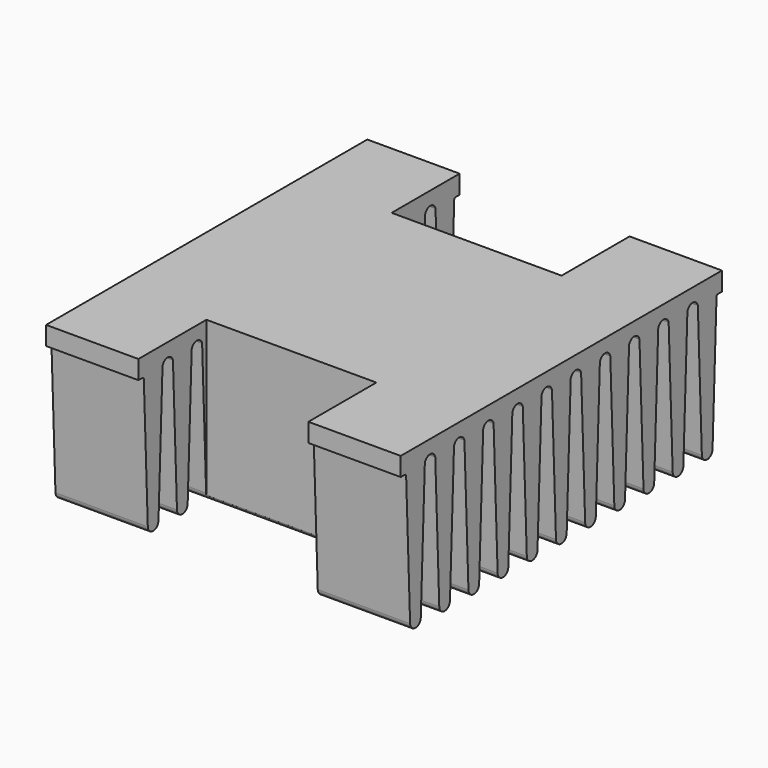
from build123d import *

# Parameters (mm, degrees)
F1_DEPTH = 130
F2_W     = 50.8
F2_H     = 25.4
F3_DEPTH = 79.5
F4_W     = 12
F4_H     = 50.7057624385
F4_H_2   = 69.7820825055
F4_H_3   = 69.8881107867
F4_H_4   = 52.3517530859
F5_DEPTH = 47.4990536315


# Not quite as in the source:
# - ends of sketch curves that miss each other by under 0.0002 mm in the source are joined
# - a feature names something its author has since deleted; it is built from what else it names


with BuildPart() as f1:
    # F0 (on Right) → F1 (new body)
    with BuildSketch(Plane.YZ):
        with BuildLine():
            Line((62.1368927236, 13.271021442), (-57.8631072764, 13.271021442))
            Line((-57.8631072764, 13.271021442), (-57.8631072764, 7.697946392))
            Line((-57.8631072764, 7.697946392), (-56.4219683785, 7.6979366796))
            ThreePointArc((-56.4219683785, 7.6979366796), (-56.0194508606, 7.5356245361), (-55.8421445251, 7.1394791077))
            Line((-55.8421445251, 7.1394791077), (-54.3616227062, -32.302053608))
            ThreePointArc((-54.3616227062, -32.302053608), (-52.3630302548, -34.2270321895), (-50.3644378034, -32.302053608))
            Line((-50.3644378034, -32.302053608), (-48.8631072764, 7.697946392))
            ThreePointArc((-48.8631072764, 7.697946392), (-46.9131019002, 9.2535299318), (-44.9631072764, 7.6979329132))
            Line((-44.9631072764, 7.6979329132), (-43.4616227062, -32.302053608))
            ThreePointArc((-43.4616227062, -32.302053608), (-41.4630302548, -34.2270321895), (-39.4644378034, -32.302053608))
            Line((-39.4644378034, -32.302053608), (-37.9631072764, 7.697946392))
            ThreePointArc((-37.9631072764, 7.697946392), (-36.0131019002, 9.2535299318), (-34.0631072764, 7.6979329132))
            Line((-34.0631072764, 7.6979329132), (-32.5616227062, -32.302053608))
            ThreePointArc((-32.5616227062, -32.302053608), (-30.5630302548, -34.2270321895), (-28.5644378034, -32.302053608))
            Line((-28.5644378034, -32.302053608), (-27.0631072764, 7.697946392))
            ThreePointArc((-27.0631072764, 7.697946392), (-25.1131019002, 9.2535299318), (-23.1631072764, 7.6979329132))
            Line((-23.1631072764, 7.6979329132), (-21.6616227062, -32.302053608))
            ThreePointArc((-21.6616227062, -32.302053608), (-19.6630302548, -34.2270321895), (-17.6644378034, -32.302053608))
            Line((-17.6644378034, -32.302053608), (-16.1631072764, 7.697946392))
            ThreePointArc((-16.1631072764, 7.697946392), (-14.2131019002, 9.2535299318), (-12.2631072764, 7.6979329132))
            Line((-12.2631072764, 7.6979329132), (-10.7616227062, -32.302053608))
            ThreePointArc((-10.7616227062, -32.302053608), (-8.7630302548, -34.2270321895), (-6.7644378034, -32.302053608))
            Line((-6.7644378034, -32.302053608), (-5.2631072764, 7.697946392))
            ThreePointArc((-5.2631072764, 7.697946392), (-3.3131019002, 9.2535299318), (-1.3631072764, 7.6979329132))
            Line((-1.3631072764, 7.6979329132), (0.1383772938, -32.302053608))
            ThreePointArc((0.1383772938, -32.302053608), (2.1369697452, -34.2270321895), (4.1355621966, -32.302053608))
            Line((4.1355621966, -32.302053608), (5.6368927236, 7.697946392))
            ThreePointArc((5.6368927236, 7.697946392), (7.5868980998, 9.2535299318), (9.5368927236, 7.6979329132))
            Line((9.5368927236, 7.6979329132), (11.0383772938, -32.302053608))
            ThreePointArc((11.0383772938, -32.302053608), (13.0369697452, -34.2270321895), (15.0355621966, -32.302053608))
            Line((15.0355621966, -32.302053608), (16.5368927236, 7.697946392))
            ThreePointArc((16.5368927236, 7.697946392), (18.4868980998, 9.2535299318), (20.4368927236, 7.6979329132))
            Line((20.4368927236, 7.6979329132), (21.9383772938, -32.302053608))
            ThreePointArc((21.9383772938, -32.302053608), (23.9369697452, -34.2270321895), (25.9355621966, -32.302053608))
            Line((25.9355621966, -32.302053608), (27.4368927236, 7.697946392))
            ThreePointArc((27.4368927236, 7.697946392), (29.3868980998, 9.2535299318), (31.3368927236, 7.6979329132))
            Line((31.3368927236, 7.6979329132), (32.8383772938, -32.302053608))
            ThreePointArc((32.8383772938, -32.302053608), (34.8369697452, -34.2270321895), (36.8355621966, -32.302053608))
            Line((36.8355621966, -32.302053608), (38.3368927236, 7.697946392))
            ThreePointArc((38.3368927236, 7.697946392), (40.2868980998, 9.2535299318), (42.2368927236, 7.6979329132))
            Line((42.2368927236, 7.6979329132), (43.7383772938, -32.302053608))
            ThreePointArc((43.7383772938, -32.302053608), (45.7369697452, -34.2270321895), (47.7355621966, -32.302053608))
            Line((47.7355621966, -32.302053608), (49.2368927236, 7.697946392))
            ThreePointArc((49.2368927236, 7.697946392), (51.1868980998, 9.2535299318), (53.1368927236, 7.6979329132))
            Line((53.1368927236, 7.6979329132), (54.6383772938, -32.302053608))
            ThreePointArc((54.6383772938, -32.302053608), (56.6369697452, -34.2270321895), (58.6355621966, -32.302053608))
            Line((58.6355621966, -32.302053608), (60.11593154, 7.1394768706))
            ThreePointArc((60.11593154, 7.1394768706), (60.2932371534, 7.5356237596), (60.6957554774, 7.697946392))
            Line((60.6957554774, 7.697946392), (62.1368927236, 7.697946392))
            Line((62.1368927236, 7.697946392), (62.1368927236, 13.271021442))
        make_face()
    extrude(amount=F1_DEPTH)

    # F2 (on face) → F3 (cut)
    with BuildSketch(Plane.XY.offset(13.271021442)):
        with Locations((65, -45.1631072764)):
            Rectangle(F2_W, F2_H)
        with Locations((65, 49.4368927236)):
            Rectangle(F2_W, F2_H)
    extrude(amount=-F3_DEPTH, mode=Mode.SUBTRACT)

    # F4 (on face) → F5 (cut, through all)
    with BuildSketch(Plane.XY.offset(13.271021442)):
        with Locations((6, 36.890672449)):
            Rectangle(F4_W, F4_H)
        with Locations((6, -23.353250023)):
            Rectangle(F4_W, F4_H_2)
        with Locations((124, -23.955682084)):
            Rectangle(F4_W, F4_H_3)
        with Locations((124, 37.1642498523)):
            Rectangle(F4_W, F4_H_4)
    extrude(amount=-F5_DEPTH, mode=Mode.SUBTRACT)


solid = f1.part
